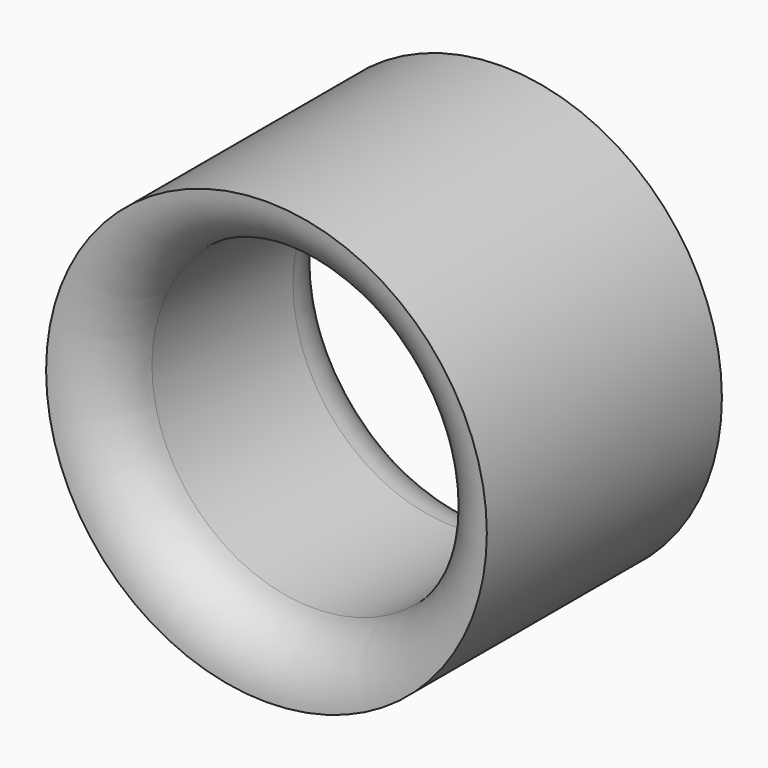
from build123d import *

# Parameters (mm, degrees)
F0_R     = 9.525
F0_R_2   = 6.985
F1_DEPTH = 12.7
F2_R     = 2.53999


# Not quite as in the source:
# - a fillet or chamfer is up to 0.001 mm smaller than in the source, because OpenCascade refuses the exact size


with BuildPart() as f1:
    # F0 (on Front) → F1 (new body)
    with BuildSketch(Plane.XZ):
        Circle(F0_R)
        Circle(F0_R_2, mode=Mode.SUBTRACT)
    extrude(amount=F1_DEPTH)

    # F2 (radius 2.54 in the source; OpenCascade refuses exactly that, so slightly less here)
    f2_edges = [f1.edges().sort_by_distance(p)[0] for p in [
        (-6.985, -12.7, 0),
        (-6.985, 0, 0),
    ]]
    fillet(f2_edges, radius=F2_R)


solid = f1.part
